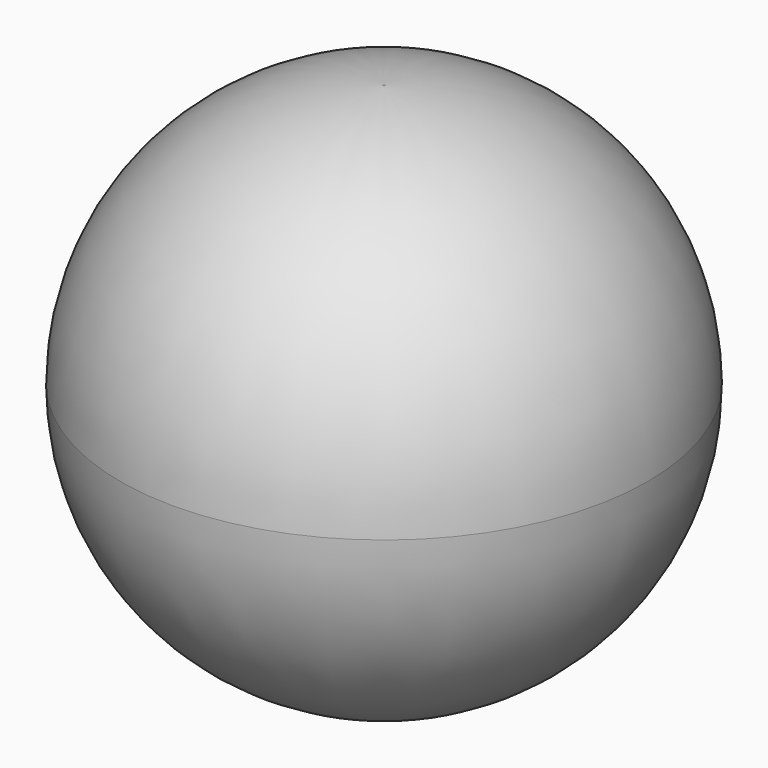
from build123d import *

# Parameters (mm, degrees)
F0_R     = 31.3645212613
F1_DEPTH = 31.242
F2_R     = 31.242
F3_R     = 31.24199


# Not quite as in the source:
# - a fillet or chamfer is up to 0.001 mm smaller than in the source, because OpenCascade refuses the exact size


with BuildPart() as f1:
    # F0 (on Top) → F1 (new body, symmetric)
    with BuildSketch(Plane.XY):
        Circle(F0_R)
    extrude(amount=F1_DEPTH, both=True)

    # F2
    f2_edges = [f1.edges().sort_by_distance(p)[0] for p in [
        (-31.364521, 0, 31.242),
    ]]
    fillet(f2_edges, radius=F2_R)

    # F3 (radius 31.242 in the source; OpenCascade refuses exactly that, so slightly less here)
    f3_edges = [f1.edges().sort_by_distance(p)[0] for p in [
        (-31.364521, 0, -31.242),
    ]]
    fillet(f3_edges, radius=F3_R)


solid = f1.part
